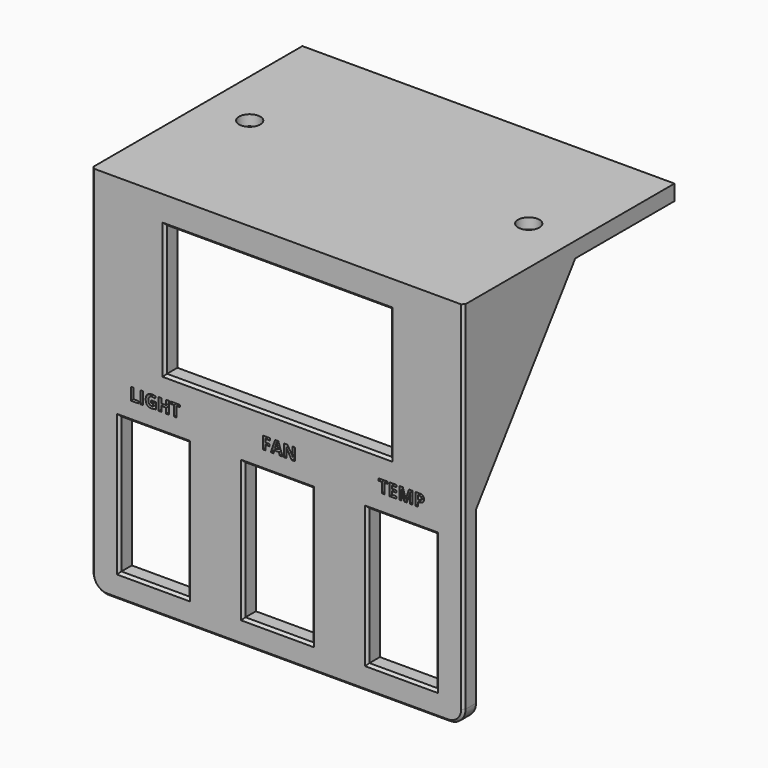
from build123d import *

# Parameters (mm, degrees)
F0_W         = 13.97
F0_H         = 27.94
F0_W_2       = 0.5341276042
F0_H_2       = 2.5185026042
F0_W_3       = 46.101
F0_H_3       = 26.797
F1_DEPTH     = 3.175
F0_TEXT_SIZE = 3.5277777778
F2_DEPTH     = 1.905
F3_W         = 76.2
F3_H         = 50.8
F3_R         = 2.1844
F4_DEPTH     = 3.175
F5_SIZE      = 1.016
F7_DEPTH     = 3.175
F9_DEPTH     = 3.175
F10_SIZE     = 0.508


# Not quite as in the source:
# - Text() gives the source's letters only with a copy of the font that has no kerning and outlines rounded to 1/6400 em; it was checked with that copy


with BuildPart() as f1:
    # F0 (on Front) → F1 (new body)
    with BuildSketch(Plane.XZ):
        with BuildLine():
            Line((38.1, 38.1), (-38.1, 38.1))
            Line((-38.1, 38.1), (-38.1, -34.925))
            ThreePointArc((-38.1, -34.925), (-37.1700640303, -37.1700640303), (-34.925, -38.1))
            Line((-34.925, -38.1), (34.925, -38.1))
            ThreePointArc((34.925, -38.1), (37.1700640303, -37.1700640303), (38.1, -34.925))
            Line((38.1, -34.925), (38.1, 38.1))
        make_face()
        with Locations((-25.4, -19.05)):
            Rectangle(F0_W, F0_H, mode=Mode.SUBTRACT)
        Polygon((-28.5045767361, -1.27), (-30.06010625, -1.27), (-30.06010625, 1.2485026042), (-29.5259786458, 1.2485026042), (-29.5259786458, -0.8290277778), (-28.5045767361, -0.8290277778), align=None, mode=Mode.SUBTRACT)
        with Locations((-27.7998480035, -0.0107486979)):
            Rectangle(F0_W_2, F0_H_2, mode=Mode.SUBTRACT)
        with BuildLine():
            Line((-25.9430793403, -0.3004123264), (-25.9430793403, 0.1444184028))
            Line((-25.9430793403, 0.1444184028), (-24.9437260417, 0.1444184028))
            Line((-24.9437260417, 0.1444184028), (-24.9437260417, -1.1614105903))
            add(Edge.make_bspline(
                [(-24.9437260417, -1.1614105903), (-25.1868119792, -1.2407855903), (-25.4012347222, -1.2727560764)],
                knots=[0, 0, 0, 1, 1, 1], degree=2))
            add(Edge.make_bspline(
                [(-25.4012347222, -1.2727560764), (-25.6156574653, -1.3047265625), (-25.8394508681, -1.3047265625)],
                knots=[0, 0, 0, 1, 1, 1], degree=2))
            add(Edge.make_bspline(
                [(-25.8394508681, -1.3047265625), (-26.4094074653, -1.3047265625), (-26.7100953993, -0.9695876736)],
                knots=[0, 0, 0, 1, 1, 1], degree=2))
            add(Edge.make_bspline(
                [(-26.7100953993, -0.9695876736), (-27.0107833333, -0.6344487847), (-27.0107833333, -0.0071657986)],
                knots=[0, 0, 0, 1, 1, 1], degree=2))
            add(Edge.make_bspline(
                [(-27.0107833333, -0.0071657986), (-27.0107833333, 0.6024782986), (-26.6618640625, 0.9434049479)],
                knots=[0, 0, 0, 1, 1, 1], degree=2))
            add(Edge.make_bspline(
                [(-26.6618640625, 0.9434049479), (-26.3129447917, 1.2843315972), (-25.6950324653, 1.2843315972)],
                knots=[0, 0, 0, 1, 1, 1], degree=2))
            add(Edge.make_bspline(
                [(-25.6950324653, 1.2843315972), (-25.3069769097, 1.2843315972), (-24.9470333333, 1.1294401042)],
                knots=[0, 0, 0, 1, 1, 1], degree=2))
            Line((-24.9470333333, 1.1294401042), (-25.1245246528, 0.7022482639))
            add(Edge.make_bspline(
                [(-25.1245246528, 0.7022482639), (-25.4001322917, 0.8400520833), (-25.6983397569, 0.8400520833)],
                knots=[0, 0, 0, 1, 1, 1], degree=2))
            add(Edge.make_bspline(
                [(-25.6983397569, 0.8400520833), (-26.0445029514, 0.8400520833), (-26.2528623264, 0.6074392361)],
                knots=[0, 0, 0, 1, 1, 1], degree=2))
            add(Edge.make_bspline(
                [(-26.2528623264, 0.6074392361), (-26.4612217014, 0.3748263889), (-26.4612217014, -0.0176388889)],
                knots=[0, 0, 0, 1, 1, 1], degree=2))
            add(Edge.make_bspline(
                [(-26.4612217014, -0.0176388889), (-26.4612217014, -0.4277430556), (-26.2933766493, -0.6438194444)],
                knots=[0, 0, 0, 1, 1, 1], degree=2))
            add(Edge.make_bspline(
                [(-26.2933766493, -0.6438194444), (-26.1255315972, -0.8598958333), (-25.8052755208, -0.8598958333)],
                knots=[0, 0, 0, 1, 1, 1], degree=2))
            add(Edge.make_bspline(
                [(-25.8052755208, -0.8598958333), (-25.6377060764, -0.8598958333), (-25.4657269097, -0.8257204861)],
                knots=[0, 0, 0, 1, 1, 1], degree=2))
            Line((-25.4657269097, -0.8257204861), (-25.4657269097, -0.3004123264))
            Line((-25.4657269097, -0.3004123264), (-25.9430793403, -0.3004123264))
        make_face(mode=Mode.SUBTRACT)
        Polygon((-22.2808050347, 1.2485026042), (-22.2808050347, -1.27), (-22.8132789931, -1.27), (-22.8132789931, -0.1830034722), (-23.8104274306, -0.1830034722), (-23.8104274306, -1.27), (-24.3445550347, -1.27), (-24.3445550347, 1.2485026042), (-23.8104274306, 1.2485026042), (-23.8104274306, 0.2612760417), (-22.8132789931, 0.2612760417), (-22.8132789931, 1.2485026042), align=None, mode=Mode.SUBTRACT)
        Polygon((-20.6734612847, 0.8042230903), (-20.6734612847, -1.27), (-21.2075888889, -1.27), (-21.2075888889, 0.8042230903), (-21.8916470486, 0.8042230903), (-21.8916470486, 1.2485026042), (-19.9899543403, 1.2485026042), (-19.9899543403, 0.8042230903), align=None, mode=Mode.SUBTRACT)
        Polygon((-2.4981076389, -0.2745052083), (-2.4981076389, -1.27), (-3.0234157986, -1.27), (-3.0234157986, 1.2485026042), (-1.5797829861, 1.2485026042), (-1.5797829861, 0.8108376736), (-2.4981076389, 0.8108376736), (-2.4981076389, 0.1615060764), (-1.6437239583, 0.1615060764), (-1.6437239583, -0.2745052083), align=None, mode=Mode.SUBTRACT)
        Polygon((1.0302213542, -1.27), (0.4547526042, -1.27), (0.2723003472, -0.6702777778), (-0.6460243056, -0.6702777778), (-0.8284765625, -1.27), (-1.4039453125, -1.27), (-0.5148350694, 1.2589756944), (0.1378038194, 1.2589756944), align=None, mode=Mode.SUBTRACT)
        with Locations((0, -19.05)):
            Rectangle(F0_W, F0_H, mode=Mode.SUBTRACT)
        with BuildLine():
            Line((3.5812456597, 1.2485026042), (3.5812456597, -1.27))
            Line((3.5812456597, -1.27), (2.9026996528, -1.27))
            Line((2.9026996528, -1.27), (1.8068836806, 0.635))
            Line((1.8068836806, 0.635), (1.7914496528, 0.635))
            add(Edge.make_bspline(
                [(1.7914496528, 0.635), (1.8245225694, 0.1306380208), (1.8245225694, -0.0848871528)],
                knots=[0, 0, 0, 1, 1, 1], degree=2))
            Line((1.8245225694, -0.0848871528), (1.8245225694, -1.27))
            Line((1.8245225694, -1.27), (1.3471701389, -1.27))
            Line((1.3471701389, -1.27), (1.3471701389, 1.2485026042))
            Line((1.3471701389, 1.2485026042), (2.0207552083, 1.2485026042))
            Line((2.0207552083, 1.2485026042), (3.1143663194, -0.6377560764))
            Line((3.1143663194, -0.6377560764), (3.1264930556, -0.6377560764))
            add(Edge.make_bspline(
                [(3.1264930556, -0.6377560764), (3.1005859375, -0.1466232639), (3.1005859375, 0.0562239583)],
                knots=[0, 0, 0, 1, 1, 1], degree=2))
            Line((3.1005859375, 0.0562239583), (3.1005859375, 1.2485026042))
            Line((3.1005859375, 1.2485026042), (3.5812456597, 1.2485026042))
        make_face(mode=Mode.SUBTRACT)
        with Locations((25.4, -19.05)):
            Rectangle(F0_W, F0_H, mode=Mode.SUBTRACT)
        Polygon((21.8723104167, 0.8042230903), (21.8723104167, -1.27), (21.3381828125, -1.27), (21.3381828125, 0.8042230903), (20.6541246528, 0.8042230903), (20.6541246528, 1.2485026042), (22.5558173611, 1.2485026042), (22.5558173611, 0.8042230903), align=None, mode=Mode.SUBTRACT)
        Polygon((24.3935690972, -0.8290277778), (24.3935690972, -1.27), (22.9433217014, -1.27), (22.9433217014, 1.2485026042), (24.3935690972, 1.2485026042), (24.3935690972, 0.8108376736), (23.4774493056, 0.8108376736), (23.4774493056, 0.25796875), (24.3301793403, 0.25796875), (24.3301793403, -0.1796961806), (23.4774493056, -0.1796961806), (23.4774493056, -0.8290277778), align=None, mode=Mode.SUBTRACT)
        with BuildLine():
            Line((26.4744067708, -1.27), (25.9849276042, -1.27))
            Line((25.9849276042, -1.27), (25.3785907986, 0.7055555556))
            Line((25.3785907986, 0.7055555556), (25.3631567708, 0.7055555556))
            add(Edge.make_bspline(
                [(25.3631567708, 0.7055555556), (25.3962296875, 0.1030772569), (25.3962296875, -0.0986675347)],
                knots=[0, 0, 0, 1, 1, 1], degree=2))
            Line((25.3962296875, -0.0986675347), (25.3962296875, -1.27))
            Line((25.3962296875, -1.27), (24.9188772569, -1.27))
            Line((24.9188772569, -1.27), (24.9188772569, 1.2485026042))
            Line((24.9188772569, 1.2485026042), (25.6459302083, 1.2485026042))
            Line((25.6459302083, 1.2485026042), (26.2417939236, -0.6774435764))
            Line((26.2417939236, -0.6774435764), (26.2522670139, -0.6774435764))
            Line((26.2522670139, -0.6774435764), (26.8845109375, 1.2485026042))
            Line((26.8845109375, 1.2485026042), (27.6110126736, 1.2485026042))
            Line((27.6110126736, 1.2485026042), (27.6110126736, -1.27))
            Line((27.6110126736, -1.27), (27.1132652778, -1.27))
            Line((27.1132652778, -1.27), (27.1132652778, -0.0777213542))
            add(Edge.make_bspline(
                [(27.1132652778, -0.0777213542), (27.1132652778, 0.0066145833), (27.1160213542, 0.1168576389)],
                knots=[0, 0, 0, 1, 1, 1], degree=2))
            add(Edge.make_bspline(
                [(27.1160213542, 0.1168576389), (27.1187774306, 0.2271006944), (27.1391723958, 0.7022482639)],
                knots=[0, 0, 0, 1, 1, 1], degree=2))
            Line((27.1391723958, 0.7022482639), (27.1237383681, 0.7022482639))
            Line((27.1237383681, 0.7022482639), (26.4744067708, -1.27))
        make_face(mode=Mode.SUBTRACT)
        with BuildLine():
            add(Edge.make_bspline(
                [(29.7461450521, 1.0511675347), (29.9845456597, 0.8538324653), (29.9845456597, 0.4630208333)],
                knots=[0, 0, 0, 1, 1, 1], degree=2))
            add(Edge.make_bspline(
                [(29.9845456597, 0.4630208333), (29.9845456597, 0.0562239583), (29.7304354167, -0.1590256076)],
                knots=[0, 0, 0, 1, 1, 1], degree=2))
            add(Edge.make_bspline(
                [(29.7304354167, -0.1590256076), (29.4763251736, -0.3742751736), (29.0077921875, -0.3742751736)],
                knots=[0, 0, 0, 1, 1, 1], degree=2))
            Line((29.0077921875, -0.3742751736), (28.7790378472, -0.3742751736))
            Line((28.7790378472, -0.3742751736), (28.7790378472, -1.27))
            Line((28.7790378472, -1.27), (28.2449102431, -1.27))
            Line((28.2449102431, -1.27), (28.2449102431, 1.2485026042))
            Line((28.2449102431, 1.2485026042), (29.0491333333, 1.2485026042))
            add(Edge.make_bspline(
                [(29.0491333333, 1.2485026042), (29.5077444444, 1.2485026042), (29.7461450521, 1.0511675347)],
                knots=[0, 0, 0, 1, 1, 1], degree=2))
        make_face(mode=Mode.SUBTRACT)
        with Locations((0, 19.05)):
            Rectangle(F0_W_3, F0_H_3, mode=Mode.SUBTRACT)
    extrude(amount=F1_DEPTH)

    # F3 (on face) → F4 (join)
    with BuildSketch(Plane.XY.offset(38.1)):
        with Locations((0, 25.4)):
            Rectangle(F3_W, F3_H)
        with Locations((-28.575, 25.4)):
            Circle(F3_R, mode=Mode.SUBTRACT)
        with Locations((28.575, 25.4)):
            Circle(F3_R, mode=Mode.SUBTRACT)
    extrude(amount=-F4_DEPTH)

    # F5
    f5_edges = [f1.edges().sort_by_distance(p)[0] for p in [
        (-30.7594, 25.4, 34.925),
        (26.3906, 25.4, 34.925),
    ]]
    chamfer(f5_edges, length=F5_SIZE)

    # F6 (on face) → F7 (join)
    with BuildSketch(Plane.YZ.offset(38.1)):
        Polygon((0, 34.925), (0, 0), (25.4, 34.925), align=None)
    extrude(amount=-F7_DEPTH)

    # F8 (on face) → F9 (join)
    with BuildSketch(Plane(origin=(-38.1, 0, 0), x_dir=(0, -1, 0), z_dir=(-1, 0, 0))):
        Polygon((-25.4, 34.925), (0, 0), (0, 34.925), align=None)
    extrude(amount=-F9_DEPTH)

    # F10
    f10_edges = [f1.edges().sort_by_distance(p)[0] for p in [
        (-23.0505, -3.175, 19.05),
        (0, -3.175, 5.6515),
        (23.0505, -3.175, 19.05),
        (0, -3.175, 32.4485),
        (32.385, -3.175, -19.05),
        (25.4, -3.175, -5.08),
        (18.415, -3.175, -19.05),
        (25.4, -3.175, -33.02),
        (6.985, -3.175, -19.05),
        (0, -3.175, -5.08),
        (-6.985, -3.175, -19.05),
        (0, -3.175, -33.02),
        (-25.4, -3.175, -33.02),
        (-32.385, -3.175, -19.05),
        (-25.4, -3.175, -5.08),
        (-18.415, -3.175, -19.05),
        (38.1, -3.175, 1.5875),
        (37.170064, -3.175, -37.170064),
        (0, -3.175, -38.1),
        (-37.170064, -3.175, -37.170064),
        (-38.1, -3.175, 1.5875),
    ]]
    chamfer(f10_edges, length=F10_SIZE)


with BuildPart() as f1b:
    # F0 (on Front) → F1, piece 2 (new body)
    with BuildSketch(Plane.XZ):
        with BuildLine():
            Line((-0.5115277778, -0.2226909722), (0.1444184028, -0.2226909722))
            add(Edge.make_bspline(
                [(0.1444184028, -0.2226909722), (-0.1085894097, 0.5920052083), (-0.1405598958, 0.6989409722)],
                knots=[0, 0, 0, 1, 1, 1], degree=2))
            add(Edge.make_bspline(
                [(-0.1405598958, 0.6989409722), (-0.1725303819, 0.8058767361), (-0.1863107639, 0.8676128472)],
                knots=[0, 0, 0, 1, 1, 1], degree=2))
            add(Edge.make_bspline(
                [(-0.1863107639, 0.8676128472), (-0.2430859375, 0.6471267361), (-0.5115277778, -0.2226909722)],
                knots=[0, 0, 0, 1, 1, 1], degree=2))
        make_face()
    extrude(amount=F1_DEPTH)


with BuildPart() as f1c:
    # F0 (on Front) → F1, piece 3 (new body)
    with BuildSketch(Plane.XZ):
        with BuildLine():
            Line((28.7790378472, 0.8108376736), (28.7790378472, 0.0633897569))
            Line((28.7790378472, 0.0633897569), (28.9548755208, 0.0633897569))
            add(Edge.make_bspline(
                [(28.9548755208, 0.0633897569), (29.2007175347, 0.0633897569), (29.3230873264, 0.1606792535)],
                knots=[0, 0, 0, 1, 1, 1], degree=2))
            add(Edge.make_bspline(
                [(29.3230873264, 0.1606792535), (29.4454571181, 0.25796875), (29.4454571181, 0.4437282986)],
                knots=[0, 0, 0, 1, 1, 1], degree=2))
            add(Edge.make_bspline(
                [(29.4454571181, 0.4437282986), (29.4454571181, 0.6316927083), (29.3429310764, 0.721265191)],
                knots=[0, 0, 0, 1, 1, 1], degree=2))
            add(Edge.make_bspline(
                [(29.3429310764, 0.721265191), (29.2404050347, 0.8108376736), (29.0215725694, 0.8108376736)],
                knots=[0, 0, 0, 1, 1, 1], degree=2))
            Line((29.0215725694, 0.8108376736), (28.7790378472, 0.8108376736))
        make_face()
    extrude(amount=F1_DEPTH)


with BuildPart() as f2:
    # F0 (on Front) → F2 (new body)
    with BuildSketch(Plane.XZ):
        with Locations((-30.3770550347, -1.27)):
            Text('LIGHT', F0_TEXT_SIZE, font='Open Sans', font_style=FontStyle.BOLD, text_align=(TextAlign.LEFT, TextAlign.BOTTOM))
        with Locations((-3.3403645833, -1.27)):
            Text('FAN', F0_TEXT_SIZE, font='Open Sans', font_style=FontStyle.BOLD, text_align=(TextAlign.LEFT, TextAlign.BOTTOM))
        with Locations((20.5835690972, -1.27)):
            Text('TEMP', F0_TEXT_SIZE, font='Open Sans', font_style=FontStyle.BOLD, text_align=(TextAlign.LEFT, TextAlign.BOTTOM))
    extrude(amount=F2_DEPTH)


solid = Compound([f1.part, f1b.part, f1c.part, f2.part])
